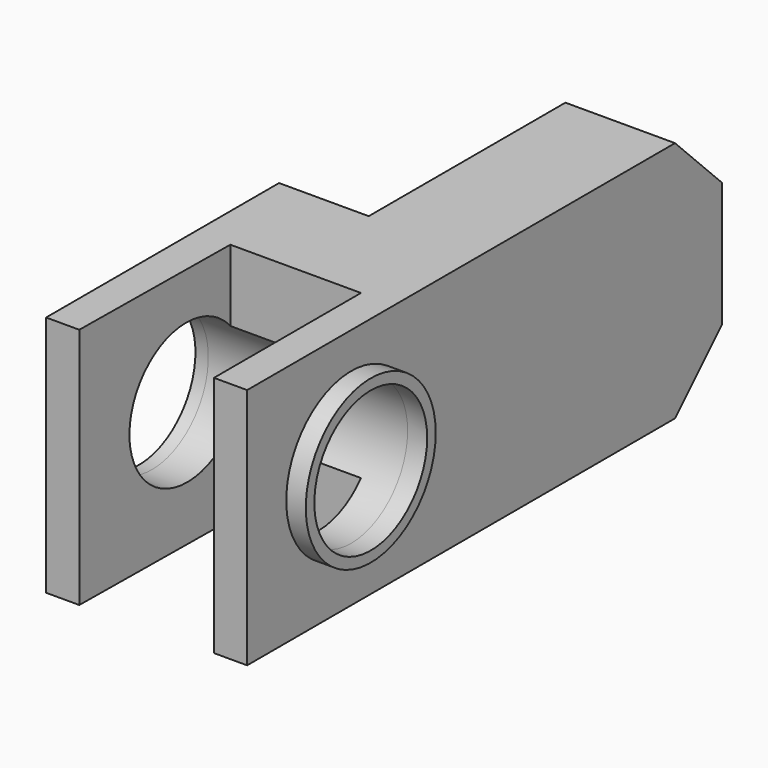
from build123d import *
from build123d import SkipClean  # not in build123d's __all__

# Parameters (mm, degrees)
F1_DEPTH = 31.496
F3_SIZE  = 7.62
F2_R     = 9.165833061
F4_DEPTH = 25.9035180712
F2_R_2   = 10.6260607341
F5_DEPTH = 1.6764
F6_R     = 10.5545569786
F6_R_2   = 9.165833061
F7_DEPTH = 2.54


with BuildPart() as f1:
    # F0 (on Top) → F1 (new body)
    with BuildSketch(Plane.XY):
        Polygon((0, 39.5732931793), (0, 0), (-11.656133458, 0), (-11.656133458, -37.8464572132), (-7.3390468024, -37.8464572132), (-7.0512411185, -13.6707741767), (9.9292984232, -13.6707741767), (9.9292984232, -37.5586524606), (14.2463846132, -37.5586524606), (14.2463846132, 0), (14.2463846132, 39.5732931793), align=None)
    extrude(amount=F1_DEPTH)

    # F3
    f3_edges = [f1.edges().sort_by_distance(p)[0] for p in [
        (7.123192, 39.573293, 31.496),
        (7.123192, 39.573293, 0),
    ]]
    chamfer(f3_edges, length=F3_SIZE)

    # F2 (on face) → F4 (cut, through all)
    with BuildSketch(Plane(origin=(-11.656133458, 0, 0), x_dir=(0, -1, 0), z_dir=(-1, 0, 0))):
        with Locations((20.6530578434, 16.2567738444)):
            Circle(F2_R)
    extrude(amount=-F4_DEPTH, mode=Mode.SUBTRACT)

    # F2 (on face) → F5 (join)
    with BuildSketch(Plane(origin=(-11.656133458, 0, 0), x_dir=(0, -1, 0), z_dir=(-1, 0, 0))):
        with Locations((20.6530578434, 16.2567738444)):
            Circle(F2_R_2)
        with Locations((20.6530578434, 16.2567738444)):
            Circle(F2_R, mode=Mode.SUBTRACT)
    extrude(amount=F5_DEPTH)

    # F6 (on face) → F7 (join)
    with BuildSketch(Plane.YZ.offset(14.2463846132)):
        with Locations((-20.6530578434, 16.2567738444)):
            Circle(F6_R)
        with Locations((-20.6530578434, 16.2567738444)):
            Circle(F6_R_2, mode=Mode.SUBTRACT)
    with SkipClean():  # cleaning this boolean's faces spoils the solid; the shape is the same uncleaned
        extrude(amount=F7_DEPTH)


solid = f1.part
